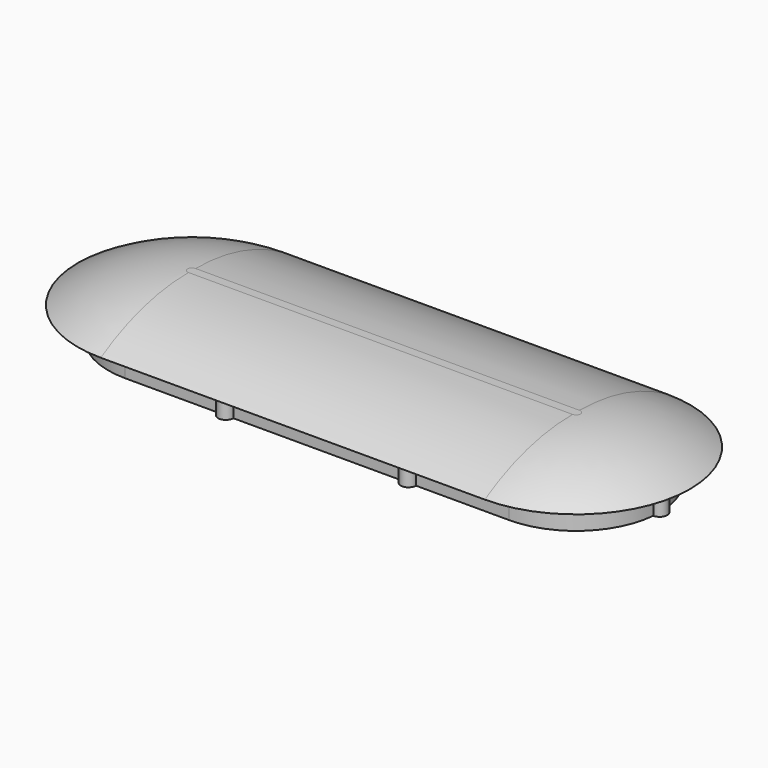
from build123d import *

# Parameters (mm, degrees)
F1_DEPTH    = 2
F2_T1_DEPTH = 25.25
F2_T4_ANGLE = 180
F2_T6_ANGLE = 180
F4_DEPTH    = 2


# Not quite as in the source:
# - a fillet or chamfer that OpenCascade refuses, or shapes differently, is made with other operations: its cross-section is extruded or revolved along the edge and cut away or added


with BuildPart() as f1:
    # F0 (on Top) → F1 (new body)
    with BuildSketch(Plane.XY):
        with BuildLine():
            Line((-12.625, -7.5), (12.625, -7.5))
            ThreePointArc((12.625, -7.5), (20.125, 0), (12.625, 7.5))
            Line((12.625, 7.5), (-12.625, 7.5))
            ThreePointArc((-12.625, 7.5), (-20.125, 0), (-12.625, -7.5))
        make_face()
    extrude(amount=F1_DEPTH)

    # F2: fillet of radius 14 on 1 edges, made by hand

    # F2_s2 → F2_t1 (cut)
    with BuildSketch(Plane.YZ.offset(-12.625)):
        with BuildLine():
            ThreePointArc((7.5, 0), (4.0305548358, 1.4907375632), (0.2888974491, 2))
            Line((0.2888974491, 2), (0.2888974491, 2.28))
            Line((0.2888974491, 2.28), (7.5, 2.28))
            Line((7.5, 2.28), (7.78, 2))
            ThreePointArc((7.78, 2), (7.78, 1), (7.644222051, 0.24))
            Line((7.644222051, 0.24), (7.5, 0))
        make_face()
        with BuildLine():
            ThreePointArc((-7.5, 0), (-4.0305548358, 1.4907375632), (-0.2888974491, 2))
            Line((-0.2888974491, 2), (-0.2888974491, 2.28))
            Line((-0.2888974491, 2.28), (-7.5, 2.28))
            Line((-7.5, 2.28), (-7.78, 2))
            ThreePointArc((-7.78, 2), (-7.78, 1), (-7.644222051, 0.24))
            Line((-7.644222051, 0.24), (-7.5, 0))
        make_face()
    extrude(amount=F2_T1_DEPTH, mode=Mode.SUBTRACT)

    # F2_s3 → F2_t4 (revolve, cut)
    with BuildSketch(Plane.YZ.offset(12.625)):
        with BuildLine():
            ThreePointArc((-7.5, 0), (-4.0305548358, 1.4907375632), (-0.2888974491, 2))
            Line((-0.2888974491, 2), (-0.2888974491, 2.28))
            Line((-0.2888974491, 2.28), (-7.5, 2.28))
            Line((-7.5, 2.28), (-7.78, 2))
            ThreePointArc((-7.78, 2), (-7.78, 1), (-7.644222051, 0.24))
            Line((-7.644222051, 0.24), (-7.5, 0))
        make_face()
    revolve(axis=Axis((12.625, 0, 2), (0, 0, 1)), revolution_arc=F2_T4_ANGLE, mode=Mode.SUBTRACT)

    # F2_s5 → F2_t6 (revolve, cut)
    with BuildSketch(Plane.YZ.offset(-12.625)):
        with BuildLine():
            ThreePointArc((7.5, 0), (4.0305548358, 1.4907375632), (0.2888974491, 2))
            Line((0.2888974491, 2), (0.2888974491, 2.28))
            Line((0.2888974491, 2.28), (7.5, 2.28))
            Line((7.5, 2.28), (7.78, 2))
            ThreePointArc((7.78, 2), (7.78, 1), (7.644222051, 0.24))
            Line((7.644222051, 0.24), (7.5, 0))
        make_face()
    revolve(axis=Axis((-12.625, 0, 2), (0, 0, 1)), revolution_arc=F2_T6_ANGLE, mode=Mode.SUBTRACT)

    # F3 (on face) → F4 (join)
    with BuildSketch(Plane(origin=(0, 0, 0), x_dir=(1, 0, 0), z_dir=(0, 0, -1))):
        with BuildLine():
            ThreePointArc((18.1022727273, 0.499483204), (16.3332908717, 4.0618442623), (12.625, 5.5))
            Line((12.625, 5.5), (6.5, 5.5))
            ThreePointArc((6.5, 5.5), (6, 6), (5.5, 5.5))
            Line((5.5, 5.5), (-5.5, 5.5))
            ThreePointArc((-5.5, 5.5), (-6, 6), (-6.5, 5.5))
            Line((-6.5, 5.5), (-12.625, 5.5))
            ThreePointArc((-12.625, 5.5), (-16.3332908717, 4.0618442623), (-18.1022727273, 0.499483204))
            ThreePointArc((-18.1022727273, 0.499483204), (-18.625, 0), (-18.1022727273, -0.499483204))
            ThreePointArc((-18.1022727273, -0.499483204), (-16.3332908717, -4.0618442623), (-12.625, -5.5))
            Line((-12.625, -5.5), (-6.5, -5.5))
            ThreePointArc((-6.5, -5.5), (-6, -6), (-5.5, -5.5))
            Line((-5.5, -5.5), (5.5, -5.5))
            ThreePointArc((5.5, -5.5), (6, -6), (6.5, -5.5))
            Line((6.5, -5.5), (12.625, -5.5))
            ThreePointArc((12.625, -5.5), (16.3332908717, -4.0618442623), (18.1022727273, -0.499483204))
            ThreePointArc((18.1022727273, -0.499483204), (18.625, 0), (18.1022727273, 0.499483204))
        make_face()
    extrude(amount=F4_DEPTH)


solid = f1.part
